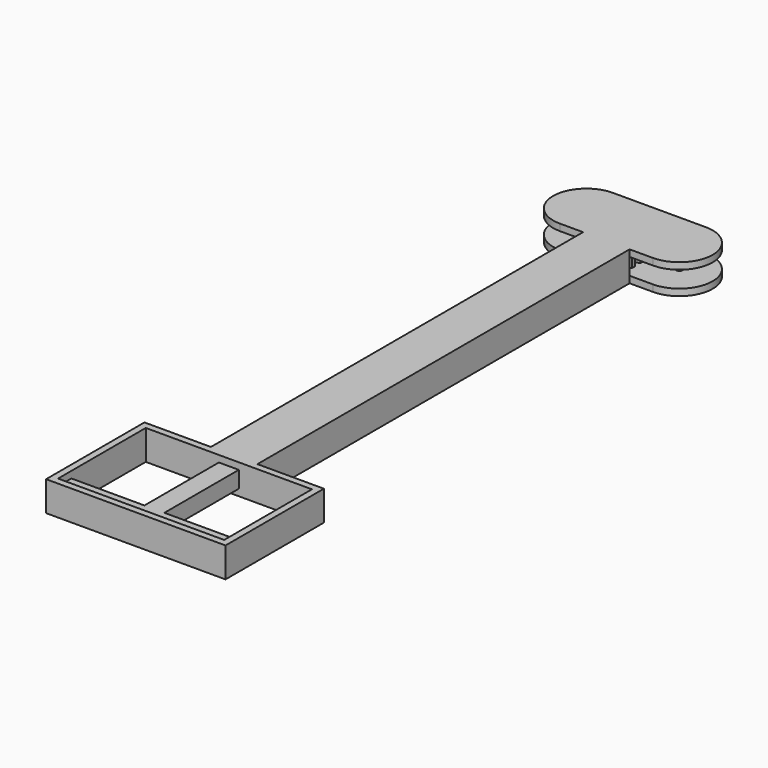
from build123d import *

# Parameters (mm, degrees)
F1_DEPTH      = 5
F3_W          = 50
F3_H          = 5
F4_DEPTH      = 5
F5_W          = 50
F5_H          = 33
F6_DEPTH      = 7
F6_DEPTH_BACK = 2
F9_DEPTH      = 5
F10_W         = 10
F10_H         = 5
F11_DEPTH     = 50
F12_R         = 1
F13_DEPTH     = 5


with BuildPart() as f1:
    # F0 (on Top) → F1 (new body)
    with BuildSketch(Plane.XY):
        Polygon((3, 13), (0, 13), (0, -180), (3, -180), (3, -39.0871235167), (3, -36.9128764833), (3, -35.8871235167), (3, -33.7128764833), (3, -32.6871235167), (3, -30.5128764833), (3, -29.4871235167), (3, -27.3128764833), (3, -26.2871235167), (3, -24.1128764833), (3, -23.0871235167), (3, -20.9128764833), (3, -19.8871235167), (3, -17.7128764833), (3, -16.6871235167), (3, -14.5128764833), (3, -13.4871235167), (3, -11.3128764833), (3, -10.2871235167), (3, -8.1128764833), (3, -7.0871235167), (3, -4.9128764833), (3, -3.8871235167), (3, -1.7128764833), (3, -0.6871235167), (3, 1.4871235167), (3, 2.5128764833), (3, 4.6871235167), (3, 5.7128764833), (3, 7.8871235167), (3, 8.9128764833), (3, 11.0871235167), align=None)
        with BuildLine():
            ThreePointArc((5, 10.5), (4.0421988802, 10.9373096378), (3, 11.0871235167))
            Line((3, 11.0871235167), (3, 8.9128764833))
            ThreePointArc((3, 8.9128764833), (4.0421988802, 9.0626903622), (5, 9.5))
            Line((5, 9.5), (5, 10))
            Line((5, 10), (5, 10.5))
        make_face()
        with BuildLine():
            Line((3, -36.9128764833), (3, -39.0871235167))
            ThreePointArc((3, -39.0871235167), (4.0421988802, -38.9373096378), (5, -38.5))
            Line((5, -38.5), (5, -38))
            Line((5, -38), (5, -37.5))
            ThreePointArc((5, -37.5), (4.0421988802, -37.0626903622), (3, -36.9128764833))
        make_face()
        with BuildLine():
            ThreePointArc((5, 7.3), (4.0421988802, 7.7373096378), (3, 7.8871235167))
            Line((3, 7.8871235167), (3, 5.7128764833))
            ThreePointArc((3, 5.7128764833), (4.0421988802, 5.8626903622), (5, 6.3))
            Line((5, 6.3), (5, 6.8))
            Line((5, 6.8), (5, 7.3))
        make_face()
        with BuildLine():
            Line((3, -33.7128764833), (3, -35.8871235167))
            ThreePointArc((3, -35.8871235167), (4.0421988802, -35.7373096378), (5, -35.3))
            Line((5, -35.3), (5, -34.8))
            Line((5, -34.8), (5, -34.3))
            ThreePointArc((5, -34.3), (4.0421988802, -33.8626903622), (3, -33.7128764833))
        make_face()
        with BuildLine():
            ThreePointArc((5, 4.1), (4.0421988802, 4.5373096378), (3, 4.6871235167))
            Line((3, 4.6871235167), (3, 2.5128764833))
            ThreePointArc((3, 2.5128764833), (4.0421988802, 2.6626903622), (5, 3.1))
            Line((5, 3.1), (5, 3.6))
            Line((5, 3.6), (5, 4.1))
        make_face()
        with BuildLine():
            Line((3, -30.5128764833), (3, -32.6871235167))
            ThreePointArc((3, -32.6871235167), (4.0421988802, -32.5373096378), (5, -32.1))
            Line((5, -32.1), (5, -31.6))
            Line((5, -31.6), (5, -31.1))
            ThreePointArc((5, -31.1), (4.0421988802, -30.6626903622), (3, -30.5128764833))
        make_face()
        with BuildLine():
            ThreePointArc((5, 0.9), (4.0421988802, 1.3373096378), (3, 1.4871235167))
            Line((3, 1.4871235167), (3, -0.6871235167))
            ThreePointArc((3, -0.6871235167), (4.0421988802, -0.5373096378), (5, -0.1))
            Line((5, -0.1), (5, 0.4))
            Line((5, 0.4), (5, 0.9))
        make_face()
        with BuildLine():
            Line((3, -27.3128764833), (3, -29.4871235167))
            ThreePointArc((3, -29.4871235167), (4.0421988802, -29.3373096378), (5, -28.9))
            Line((5, -28.9), (5, -28.4))
            Line((5, -28.4), (5, -27.9))
            ThreePointArc((5, -27.9), (4.0421988802, -27.4626903622), (3, -27.3128764833))
        make_face()
        with BuildLine():
            ThreePointArc((5, -2.3), (4.0421988802, -1.8626903622), (3, -1.7128764833))
            Line((3, -1.7128764833), (3, -3.8871235167))
            ThreePointArc((3, -3.8871235167), (4.0421988802, -3.7373096378), (5, -3.3))
            Line((5, -3.3), (5, -2.8))
            Line((5, -2.8), (5, -2.3))
        make_face()
        with BuildLine():
            Line((3, -24.1128764833), (3, -26.2871235167))
            ThreePointArc((3, -26.2871235167), (4.0421988802, -26.1373096378), (5, -25.7))
            Line((5, -25.7), (5, -25.2))
            Line((5, -25.2), (5, -24.7))
            ThreePointArc((5, -24.7), (4.0421988802, -24.2626903622), (3, -24.1128764833))
        make_face()
        with BuildLine():
            ThreePointArc((5, -5.5), (4.0421988802, -5.0626903622), (3, -4.9128764833))
            Line((3, -4.9128764833), (3, -7.0871235167))
            ThreePointArc((3, -7.0871235167), (4.0421988802, -6.9373096378), (5, -6.5))
            Line((5, -6.5), (5, -6))
            Line((5, -6), (5, -5.5))
        make_face()
        with BuildLine():
            Line((3, -20.9128764833), (3, -23.0871235167))
            ThreePointArc((3, -23.0871235167), (4.0421988802, -22.9373096378), (5, -22.5))
            Line((5, -22.5), (5, -22))
            Line((5, -22), (5, -21.5))
            ThreePointArc((5, -21.5), (4.0421988802, -21.0626903622), (3, -20.9128764833))
        make_face()
        with BuildLine():
            ThreePointArc((5, -8.7), (4.0421988802, -8.2626903622), (3, -8.1128764833))
            Line((3, -8.1128764833), (3, -10.2871235167))
            ThreePointArc((3, -10.2871235167), (4.0421988802, -10.1373096378), (5, -9.7))
            Line((5, -9.7), (5, -9.2))
            Line((5, -9.2), (5, -8.7))
        make_face()
        with BuildLine():
            Line((3, -17.7128764833), (3, -19.8871235167))
            ThreePointArc((3, -19.8871235167), (4.0421988802, -19.7373096378), (5, -19.3))
            Line((5, -19.3), (5, -18.8))
            Line((5, -18.8), (5, -18.3))
            ThreePointArc((5, -18.3), (4.0421988802, -17.8626903622), (3, -17.7128764833))
        make_face()
        with BuildLine():
            ThreePointArc((5, -11.9), (4.0421988802, -11.4626903622), (3, -11.3128764833))
            Line((3, -11.3128764833), (3, -13.4871235167))
            ThreePointArc((3, -13.4871235167), (4.0421988802, -13.3373096378), (5, -12.9))
            Line((5, -12.9), (5, -12.4))
            Line((5, -12.4), (5, -11.9))
        make_face()
        with BuildLine():
            Line((3, -14.5128764833), (3, -16.6871235167))
            ThreePointArc((3, -16.6871235167), (4.0421988802, -16.5373096378), (5, -16.1))
            Line((5, -16.1), (5, -15.6))
            Line((5, -15.6), (5, -15.1))
            ThreePointArc((5, -15.1), (4.0421988802, -14.6626903622), (3, -14.5128764833))
        make_face()
    extrude(amount=F1_DEPTH)

    # F2: F1 across face


with BuildPart() as f1_1:
    add(f1.part)
    add(f1.part.mirror(Plane(origin=(0, -83.5, 2.5), x_dir=(0, -1, 0), z_dir=(-1, 0, 0))))

    # F3 (on face) → F4 (join)
    with BuildSketch(Plane.XZ.offset(180)):
        with Locations((0, 2.5)):
            Rectangle(F3_W, F3_H)
    extrude(amount=F4_DEPTH)


with BuildPart() as f6:
    # F5 (on Top) → F6 (new body, two sides)
    with BuildSketch(Plane.XY) as f6_sk:
        with BuildLine():
            ThreePointArc((14, -10), (21.0710678119, -7.0710678119), (24, 0))
            ThreePointArc((24, 0), (21.0710678119, 7.0710678119), (14, 10))
            ThreePointArc((14, 10), (4, 0), (14, -10))
        make_face()
        with BuildLine():
            ThreePointArc((14, -10), (4, 0), (14, 10))
            Line((14, 10), (0, 10))
            Line((0, 10), (-14, 10))
            ThreePointArc((-14, 10), (-6.9289321881, 7.0710678119), (-4, 0))
            ThreePointArc((-4, 0), (-6.9289321881, -7.0710678119), (-14, -10))
            Line((-14, -10), (-7, -10))
            Line((-7, -10), (-7, -150))
            Line((-7, -150), (-27, -150))
            Line((-27, -150), (-27, -187))
            Line((-27, -187), (0, -187))
            Line((0, -187), (27, -187))
            Line((27, -187), (27, -150))
            Line((27, -150), (7, -150))
            Line((7, -150), (7, -10))
            Line((7, -10), (14, -10))
        make_face()
        with Locations((0, -168.5)):
            Rectangle(F5_W, F5_H, mode=Mode.SUBTRACT)
        with BuildLine():
            ThreePointArc((-4, 0), (-6.9289321881, 7.0710678119), (-14, 10))
            ThreePointArc((-14, 10), (-24, 0), (-14, -10))
            ThreePointArc((-14, -10), (-6.9289321881, -7.0710678119), (-4, 0))
        make_face()
    extrude(amount=F6_DEPTH)
    extrude(f6_sk.sketch, amount=-F6_DEPTH_BACK)

    # F7: cut F1
    add(f1_1.part, mode=Mode.SUBTRACT)

    # F8 (on Top) → F9 (cut)
    with BuildSketch(Plane.XY):
        with BuildLine():
            ThreePointArc((-14, 10), (-24, 0), (-14, -10))
            Line((-14, -10), (14, -10))
            ThreePointArc((14, -10), (24, 0), (14, 10))
            Line((14, 10), (-14, 10))
        make_face()
    extrude(amount=F9_DEPTH, mode=Mode.SUBTRACT)

    # F10 (on face) → F11 (cut)
    with BuildSketch(Plane(origin=(0, -10, 0), x_dir=(-1, 0, 0), z_dir=(0, 1, 0))):
        with Locations((0, 2.5)):
            Rectangle(F10_W, F10_H)
    extrude(amount=-F11_DEPTH, mode=Mode.SUBTRACT)

    # F12 (on Top) → F13 (join, through all)
    with BuildSketch(Plane.XY):
        with Locations((-14, 0)):
            Circle(F12_R)
        with Locations((14, 0)):
            Circle(F12_R)
    extrude(amount=F13_DEPTH)


solid = Compound([f1_1.part, f6.part])
